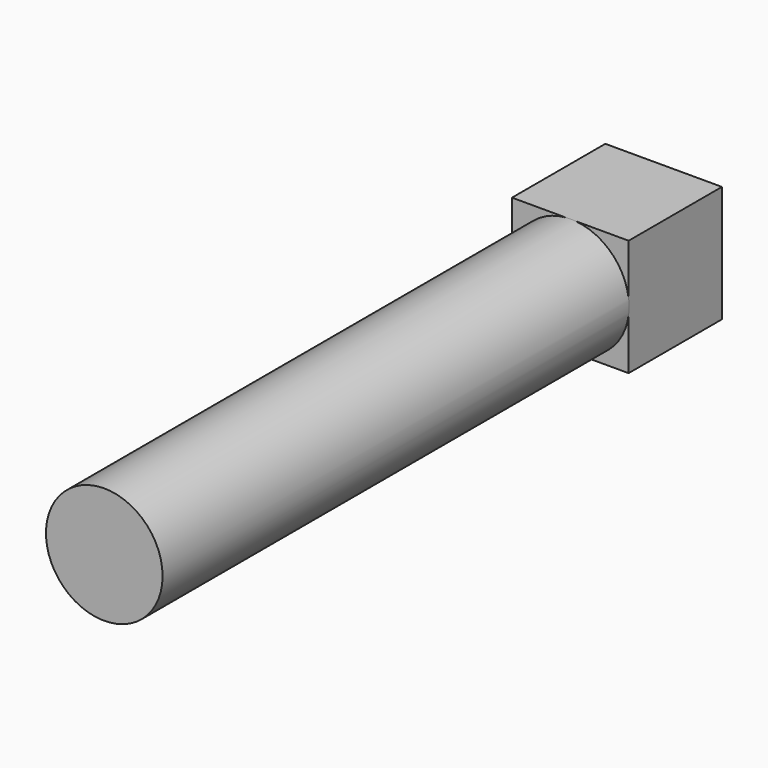
from build123d import *

# Parameters (mm, degrees)
F0_R     = 12.7
F1_DEPTH = 127
F5_DEPTH = 25.4


# Not quite as in the source:
# - the program builds the solid bodies; features that only make, move or delete a surface that nothing else refers to are left out


with BuildPart() as f1:
    # F0 (on Front) → F1 (new body)
    with BuildSketch(Plane.XZ):
        with Locations((48.1354147196, 27.8021357954)):
            Circle(F0_R)
    extrude(amount=F1_DEPTH)

    # F2 (on face) → F5 (join)
    with BuildSketch(Plane(origin=(0, 0, 0), x_dir=(-1, 0, 0), z_dir=(0, 1, 0))):
        with BuildLine():
            Line((-49.2203550876, 40.4557085872), (-60.73924371, 40.4557085872))
            Line((-60.73924371, 40.4557085872), (-60.73924371, 29.3621020704))
            ThreePointArc((-60.73924371, 29.3621020704), (-56.94521767, 36.9496694507), (-49.2203550876, 40.4557085872))
        make_face()
        with BuildLine():
            Line((-35.33924371, 40.4557085872), (-47.0504743515, 40.4557085872))
            ThreePointArc((-47.0504743515, 40.4557085872), (-38.7794342078, 36.3902455212), (-35.4354147196, 27.8021357954))
            ThreePointArc((-35.4354147196, 27.8021357954), (-47.3539507661, 15.126201349), (-60.73924371, 26.2421695203))
            Line((-60.73924371, 26.2421695203), (-60.73924371, 15.0557085872))
            Line((-60.73924371, 15.0557085872), (-35.33924371, 15.0557085872))
            Line((-35.33924371, 15.0557085872), (-35.33924371, 40.4557085872))
        make_face()
        with BuildLine():
            Line((-47.0504743515, 40.4557085872), (-49.2203550876, 40.4557085872))
            ThreePointArc((-49.2203550876, 40.4557085872), (-56.94521767, 36.9496694507), (-60.73924371, 29.3621020704))
            Line((-60.73924371, 29.3621020704), (-60.73924371, 26.2421695203))
            ThreePointArc((-60.73924371, 26.2421695203), (-47.3539507661, 15.126201349), (-35.4354147196, 27.8021357954))
            ThreePointArc((-35.4354147196, 27.8021357954), (-38.7794342078, 36.3902455212), (-47.0504743515, 40.4557085872))
        make_face()
    extrude(amount=F5_DEPTH)


solid = f1.part
